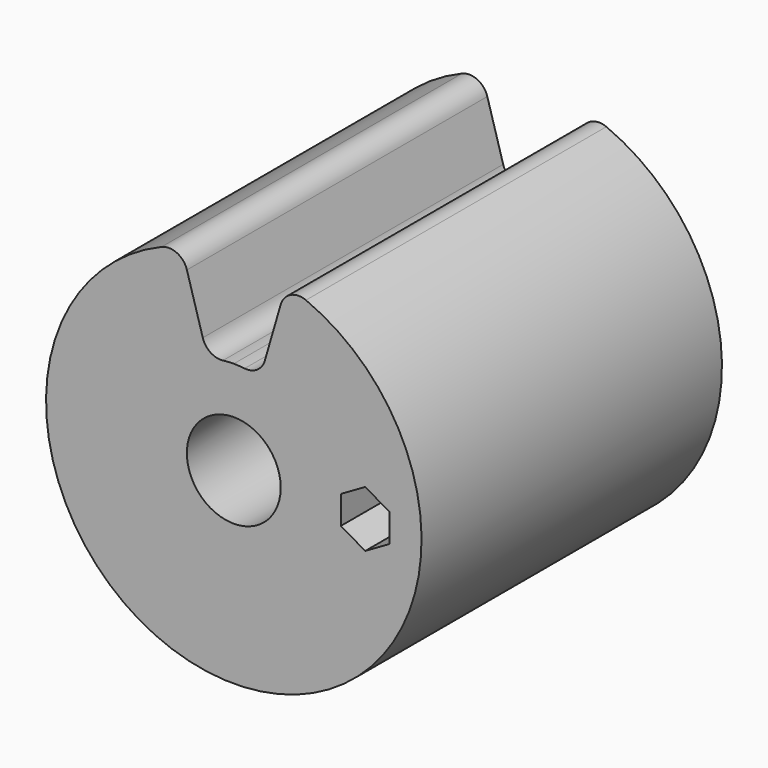
from build123d import *

# Parameters (mm, degrees)
F0_R      = 10
F1_DEPTH  = 20
F2_R      = 2.5
F3_DEPTH  = 5
F13_DEPTH = 20.001
F4_R      = 1
F6_DEPTH  = 20.001
F9_R      = 5.3210242514
F10_DEPTH = 25


# Not quite as in the source:
# - the program builds the solid bodies; features that only make, move or delete a surface that nothing else refers to are left out


with BuildPart() as f1:
    # F0 (on Front) → F1 (new body)
    with BuildSketch(Plane.XZ):
        Circle(F0_R)
    extrude(amount=F1_DEPTH)

    # F2 (on face) → F3 (cut)
    with BuildSketch(Plane.XZ.offset(20)):
        Circle(F2_R)
    extrude(amount=-F3_DEPTH, mode=Mode.SUBTRACT)

    # F12 (on face) → F13 (cut, through all)
    with BuildSketch(Plane.XZ.offset(20)):
        with BuildLine():
            ThreePointArc((2.7924241272, 9.6022063868), (1.4103077913, 9.9000521177), (0, 10))
            Line((0, 10), (0, 5))
            ThreePointArc((0, 5), (0.7051538957, 4.9500260589), (1.3962120636, 4.8011031934))
            Line((1.3962120636, 4.8011031934), (2.7924241272, 9.6022063868))
        make_face()
        with BuildLine():
            Line((0, 5), (0, 10))
            ThreePointArc((0, 10), (-1.4103077913, 9.9000521177), (-2.7924241272, 9.6022063868))
            Line((-2.7924241272, 9.6022063868), (-1.3962120636, 4.8011031934))
            ThreePointArc((-1.3962120636, 4.8011031934), (-0.7051538957, 4.9500260589), (0, 5))
        make_face()
    extrude(amount=-F13_DEPTH, mode=Mode.SUBTRACT)

    # F4
    f4_edges = [f1.edges().sort_by_distance(p)[0] for p in [
        (-2.792424, -10, 9.602206),
        (2.792424, -10, 9.602206),
        (-1.396212, -10, 4.801103),
        (1.396212, -10, 4.801103),
    ]]
    fillet(f4_edges, radius=F4_R)

    # F5 (on face) → F6 (cut, through all)
    with BuildSketch(Plane.XZ.offset(20)):
        Polygon((8.2990381057, 0.75), (7, 1.5), (5.7009618943, 0.75), (5.7009618943, -0.75), (7, -1.5), (8.2990381057, -0.75), align=None)
    extrude(amount=-F6_DEPTH, mode=Mode.SUBTRACT)

    # F9 (on face) → F10 (cut)
    with BuildSketch(Plane(origin=(0, 0, 0), x_dir=(-1, 0, 0), z_dir=(0, 1, 0))):
        with Locations((11.770372279, -20.3817021102)):
            Circle(F9_R)
    extrude(amount=-F10_DEPTH, mode=Mode.SUBTRACT)


solid = f1.part
